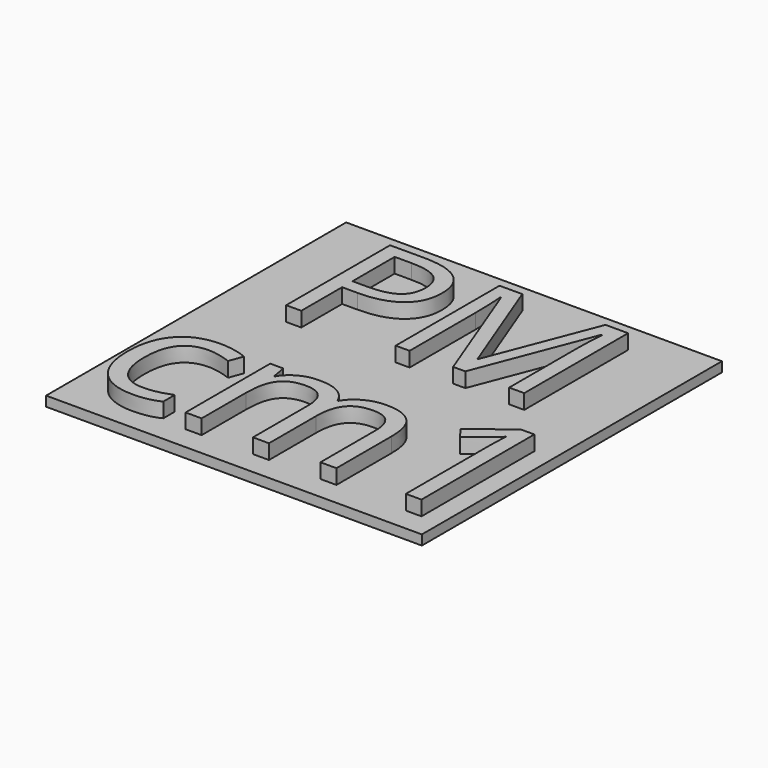
from build123d import *

# Parameters (mm, degrees)
F0_W           = 76.366558671
F0_H           = 76.2208253145
F1_DEPTH       = 2
F2_TEXT_SIZE   = 36.9559093896
F2_TEXT_SIZE_2 = 40.1694689774
F3_DEPTH       = 3


# Not quite as in the source:
# - Text() gives the source's letters only with a copy of the font that has no kerning and outlines rounded to 1/6400 em; it was checked with that copy


with BuildPart() as f1:
    # F0 (on Top) → F1 (new body)
    with BuildSketch(Plane.XY):
        with Locations((-38.1832793355, 38.1104126573)):
            Rectangle(F0_W, F0_H)
    extrude(amount=F1_DEPTH)

    # F2 (on face) → F3 (join)
    with BuildSketch(Plane.XY.offset(2)):
        with Locations((-66.047033295, 43.5596033931)):
            Text('PM', F2_TEXT_SIZE, font='Open Sans', text_align=(TextAlign.LEFT, TextAlign.BOTTOM))
        with Locations((-74.4352380279, 4.8041008413)):
            Text('cm1', F2_TEXT_SIZE_2, font='Open Sans', text_align=(TextAlign.LEFT, TextAlign.BOTTOM))
    extrude(amount=F3_DEPTH)


solid = f1.part
